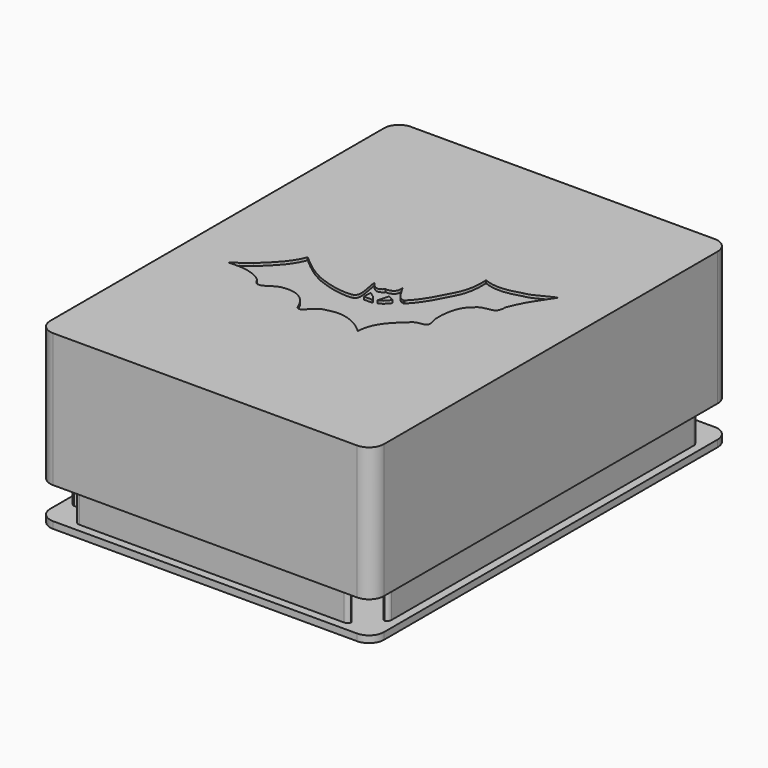
from build123d import *

# Parameters (mm, degrees)
F1_W        = 1.5
F1_H        = 85.4
F1_W_2      = 60.4
F1_H_2      = 1.5
F2_DEPTH    = 1.5
F3_DEPTH    = 29.5
F4_T1_DEPTH = 30.5
F5_DEPTH    = 29.5
F7_T        = -1.5
F9_DEPTH    = 0.6


# Not quite as in the source:
# - a fillet or chamfer that OpenCascade refuses, or shapes differently, is made with other operations: its cross-section is extruded or revolved along the edge and cut away or added


with BuildPart() as f2:
    # F1 (on Top) → F2 (new body)
    with BuildSketch(Plane.XY):
        with BuildLine():
            Line((-35, -46), (-35, -43.0606123087))
            ThreePointArc((-35, -43.0606123087), (-36.3142494559, -44.276631206), (-36.8, -46))
            ThreePointArc((-36.8, -46), (-35.8334523867, -48.3334523691), (-33.5000000248, -49.3))
            ThreePointArc((-33.5000000248, -49.3), (-31.7766312166, -48.8142494624), (-30.5606123087, -47.5))
            Line((-30.5606123087, -47.5), (-33.5000000271, -47.5))
            Line((-33.5000000271, -47.5), (-35, -47.5))
            Line((-35, -47.5), (-35, -46))
        make_face()
        with BuildLine():
            ThreePointArc((33.5, 42.7), (31.1665476221, 43.6665476221), (30.2, 46))
            Line((30.2, 46), (-30.2, 46))
            ThreePointArc((-30.2, 46), (-31.1665476221, 43.6665476221), (-33.5, 42.7))
            Line((-33.5, 42.7), (-33.5, -42.7))
            ThreePointArc((-33.5, -42.7), (-31.1665476221, -43.6665476221), (-30.2, -46))
            Line((-30.2, -46), (30.2, -46))
            ThreePointArc((30.2, -46), (31.1665476221, -43.6665476221), (33.5, -42.7))
            Line((33.5, -42.7), (33.5, 42.7))
        make_face()
        with Locations((34.25, 0)):
            Rectangle(F1_W, F1_H)
        with Locations((-34.25, 0)):
            Rectangle(F1_W, F1_H)
        with BuildLine():
            ThreePointArc((36.8, 46), (36.3142494559, 44.276631206), (35, 43.0606123087))
            Line((35, 43.0606123087), (35, 42.7))
            Line((35, 42.7), (35, -42.7))
            Line((35, -42.7), (35, -43.0606123087))
            ThreePointArc((35, -43.0606123087), (36.3142494559, -44.276631206), (36.8, -46))
            Line((36.8, -46), (36.8, 46))
        make_face()
        with BuildLine():
            ThreePointArc((33.5, -49.3), (31.776631206, -48.8142494559), (30.5606123087, -47.5))
            Line((30.5606123087, -47.5), (30.2, -47.5))
            Line((30.2, -47.5), (-30.2, -47.5))
            Line((-30.2, -47.5), (-30.5606123087, -47.5))
            ThreePointArc((-30.5606123087, -47.5), (-31.7766312166, -48.8142494624), (-33.5000000248, -49.3))
            Line((-33.5000000248, -49.3), (33.5, -49.3))
        make_face()
        with Locations((0, 46.75)):
            Rectangle(F1_W_2, F1_H_2)
        with BuildLine():
            Line((32, 46), (30.2, 46))
            ThreePointArc((30.2, 46), (31.1665476221, 43.6665476221), (33.5, 42.7))
            Line((33.5, 42.7), (33.5, 44.5))
            ThreePointArc((33.5, 44.5), (32.4393398282, 44.9393398282), (32, 46))
        make_face()
        with BuildLine():
            ThreePointArc((33.5, 49.3), (31.776631206, 48.8142494559), (30.5606123087, 47.5))
            Line((30.5606123087, 47.5), (33.5, 47.5))
            Line((33.5, 47.5), (35, 47.5))
            Line((35, 47.5), (35, 46))
            Line((35, 46), (35, 43.0606123087))
            ThreePointArc((35, 43.0606123087), (36.3142494559, 44.276631206), (36.8, 46))
            ThreePointArc((36.8, 46), (35.8334523779, 48.3334523779), (33.5, 49.3))
        make_face()
        with Locations((0, -46.75)):
            Rectangle(F1_W_2, F1_H_2)
        with BuildLine():
            Line((-33.4999999666, 47.5), (-30.5606123087, 47.5))
            ThreePointArc((-30.5606123087, 47.5), (-31.776631206, 48.8142494559), (-33.5, 49.3))
            ThreePointArc((-33.5, 49.3), (-35.8334523779, 48.3334523779), (-36.8, 46))
            ThreePointArc((-36.8, 46), (-36.3142494559, 44.276631206), (-35, 43.0606123087))
            Line((-35, 43.0606123087), (-35, 46))
            Line((-35, 46), (-35, 47.5))
            Line((-35, 47.5), (-33.4999999666, 47.5))
        make_face()
        with BuildLine():
            Line((33.5, -44.5), (33.5, -42.7))
            ThreePointArc((33.5, -42.7), (31.1665476221, -43.6665476221), (30.2, -46))
            Line((30.2, -46), (32, -46))
            ThreePointArc((32, -46), (32.4393398282, -44.9393398282), (33.5, -44.5))
        make_face()
        with BuildLine():
            Line((-35, 42.7), (-35, 43.0606123087))
            ThreePointArc((-35, 43.0606123087), (-36.3142494559, 44.276631206), (-36.8, 46))
            Line((-36.8, 46), (-36.8, -46))
            ThreePointArc((-36.8, -46), (-36.3142494559, -44.276631206), (-35, -43.0606123087))
            Line((-35, -43.0606123087), (-35, -42.7))
            Line((-35, -42.7), (-35, 42.7))
        make_face()
        with BuildLine():
            ThreePointArc((-33.5, 42.7), (-31.1665476221, 43.6665476221), (-30.2, 46))
            Line((-30.2, 46), (-32, 46))
            ThreePointArc((-32, 46), (-32.4393398282, 44.9393398282), (-33.5, 44.5))
            Line((-33.5, 44.5), (-33.5, 42.7))
        make_face()
        with BuildLine():
            ThreePointArc((-30.2, -46), (-31.1665476221, -43.6665476221), (-33.5, -42.7))
            Line((-33.5, -42.7), (-33.5, -44.5))
            ThreePointArc((-33.5, -44.5), (-32.4393398282, -44.9393398282), (-32, -46))
            Line((-32, -46), (-30.2, -46))
        make_face()
        with BuildLine():
            Line((30.2, 47.5), (30.5606123087, 47.5))
            ThreePointArc((30.5606123087, 47.5), (31.776631206, 48.8142494559), (33.5, 49.3))
            Line((33.5, 49.3), (-33.5, 49.3))
            ThreePointArc((-33.5, 49.3), (-31.776631206, 48.8142494559), (-30.5606123087, 47.5))
            Line((-30.5606123087, 47.5), (-30.2, 47.5))
            Line((-30.2, 47.5), (30.2, 47.5))
        make_face()
        with BuildLine():
            Line((-32, 46), (-30.2, 46))
            ThreePointArc((-30.2, 46), (-30.2914193651, 46.7713691135), (-30.5606123087, 47.5))
            Line((-30.5606123087, 47.5), (-33.4999999666, 47.5))
            ThreePointArc((-33.4999999666, 47.5), (-32.4393398164, 47.06066016), (-32, 46))
        make_face()
        with BuildLine():
            ThreePointArc((36.8, -46), (36.3142494559, -44.276631206), (35, -43.0606123087))
            Line((35, -43.0606123087), (35, -46))
            Line((35, -46), (35, -47.5))
            Line((35, -47.5), (33.5, -47.5))
            Line((33.5, -47.5), (30.5606123087, -47.5))
            ThreePointArc((30.5606123087, -47.5), (31.776631206, -48.8142494559), (33.5, -49.3))
            ThreePointArc((33.5, -49.3), (35.8334523779, -48.3334523779), (36.8, -46))
        make_face()
        with BuildLine():
            ThreePointArc((33.5, 47.5), (32.4393398282, 47.0606601718), (32, 46))
            Line((32, 46), (33.5, 46))
            Line((33.5, 46), (33.5, 44.5))
            ThreePointArc((33.5, 44.5), (34.5606601718, 44.9393398282), (35, 46))
            ThreePointArc((35, 46), (34.5606601718, 47.0606601718), (33.5, 47.5))
        make_face()
        with BuildLine():
            ThreePointArc((-30.5606123087, -47.5), (-30.2914193651, -46.7713691135), (-30.2, -46))
            Line((-30.2, -46), (-32, -46))
            ThreePointArc((-32, -46), (-32.4393398378, -47.0606601813), (-33.5000000271, -47.5))
            Line((-33.5000000271, -47.5), (-30.5606123087, -47.5))
        make_face()
        with BuildLine():
            ThreePointArc((35, -43.0606123087), (34.2713691135, -42.7914193651), (33.5, -42.7))
            Line((33.5, -42.7), (33.5, -44.5))
            ThreePointArc((33.5, -44.5), (34.5606601718, -44.9393398282), (35, -46))
            Line((35, -46), (35, -43.0606123087))
        make_face()
        with BuildLine():
            ThreePointArc((30.5606123087, 47.5), (30.2914193651, 46.7713691135), (30.2, 46))
            Line((30.2, 46), (32, 46))
            ThreePointArc((32, 46), (32.4393398282, 47.0606601718), (33.5, 47.5))
            Line((33.5, 47.5), (30.5606123087, 47.5))
        make_face()
        with BuildLine():
            Line((-33.5, 46), (-32, 46))
            ThreePointArc((-32, 46), (-32.4393398164, 47.06066016), (-33.4999999666, 47.5))
            ThreePointArc((-33.4999999666, 47.5), (-34.56066016, 47.0606601836), (-35, 46))
            ThreePointArc((-35, 46), (-34.5606601718, 44.9393398282), (-33.5, 44.5))
            Line((-33.5, 44.5), (-33.5, 46))
        make_face()
        with BuildLine():
            Line((32, -46), (30.2, -46))
            ThreePointArc((30.2, -46), (30.2914193651, -46.7713691135), (30.5606123087, -47.5))
            Line((30.5606123087, -47.5), (33.5, -47.5))
            ThreePointArc((33.5, -47.5), (32.4393398282, -47.0606601718), (32, -46))
        make_face()
        with BuildLine():
            ThreePointArc((35, 43.0606123087), (34.2713691135, 42.7914193651), (33.5, 42.7))
            Line((33.5, 42.7), (35, 42.7))
            Line((35, 42.7), (35, 43.0606123087))
        make_face()
        with BuildLine():
            ThreePointArc((-32, -46), (-32.4393398282, -44.9393398282), (-33.5, -44.5))
            Line((-33.5, -44.5), (-33.5, -46))
            Line((-33.5, -46), (-32, -46))
        make_face()
        with BuildLine():
            Line((33.5, -46), (33.5, -44.5))
            ThreePointArc((33.5, -44.5), (32.4393398282, -44.9393398282), (32, -46))
            Line((32, -46), (33.5, -46))
        make_face()
        with BuildLine():
            Line((-33.5, -44.5), (-33.5, -42.7))
            ThreePointArc((-33.5, -42.7), (-34.2713691135, -42.7914193651), (-35, -43.0606123087))
            Line((-35, -43.0606123087), (-35, -46))
            ThreePointArc((-35, -46), (-34.5606601718, -44.9393398282), (-33.5, -44.5))
        make_face()
        with BuildLine():
            ThreePointArc((-35, 43.0606123087), (-34.2713691135, 42.7914193651), (-33.5, 42.7))
            Line((-33.5, 42.7), (-33.5, 44.5))
            ThreePointArc((-33.5, 44.5), (-34.5606601718, 44.9393398282), (-35, 46))
            Line((-35, 46), (-35, 43.0606123087))
        make_face()
        with BuildLine():
            Line((-33.5, -46), (-33.5, -44.5))
            ThreePointArc((-33.5, -44.5), (-34.5606601718, -44.9393398282), (-35, -46))
            ThreePointArc((-35, -46), (-34.5606601813, -47.0606601622), (-33.5000000271, -47.5))
            ThreePointArc((-33.5000000271, -47.5), (-32.4393398378, -47.0606601813), (-32, -46))
            Line((-32, -46), (-33.5, -46))
        make_face()
        with BuildLine():
            Line((33.5, 44.5), (33.5, 42.7))
            ThreePointArc((33.5, 42.7), (34.2713691135, 42.7914193651), (35, 43.0606123087))
            Line((35, 43.0606123087), (35, 46))
            ThreePointArc((35, 46), (34.5606601718, 44.9393398282), (33.5, 44.5))
        make_face()
        with BuildLine():
            Line((-30.2, -47.5), (-30.2, -46))
            ThreePointArc((-30.2, -46), (-30.2914193651, -46.7713691135), (-30.5606123087, -47.5))
            Line((-30.5606123087, -47.5), (-30.2, -47.5))
        make_face()
        with BuildLine():
            ThreePointArc((-30.5606123087, 47.5), (-30.2914193651, 46.7713691135), (-30.2, 46))
            Line((-30.2, 46), (-30.2, 47.5))
            Line((-30.2, 47.5), (-30.5606123087, 47.5))
        make_face()
        with BuildLine():
            Line((30.2, 47.5), (30.2, 46))
            ThreePointArc((30.2, 46), (30.2914193651, 46.7713691135), (30.5606123087, 47.5))
            Line((30.5606123087, 47.5), (30.2, 47.5))
        make_face()
        with BuildLine():
            ThreePointArc((-35, -43.0606123087), (-34.2713691135, -42.7914193651), (-33.5, -42.7))
            Line((-33.5, -42.7), (-35, -42.7))
            Line((-35, -42.7), (-35, -43.0606123087))
        make_face()
        with BuildLine():
            Line((33.5, 46), (32, 46))
            ThreePointArc((32, 46), (32.4393398282, 44.9393398282), (33.5, 44.5))
            Line((33.5, 44.5), (33.5, 46))
        make_face()
        with BuildLine():
            ThreePointArc((-35, 46), (-34.56066016, 47.0606601836), (-33.4999999666, 47.5))
            Line((-33.4999999666, 47.5), (-35, 47.5))
            Line((-35, 47.5), (-35, 46))
        make_face()
        with BuildLine():
            ThreePointArc((-33.5000000271, -47.5), (-34.5606601813, -47.0606601622), (-35, -46))
            Line((-35, -46), (-35, -47.5))
            Line((-35, -47.5), (-33.5000000271, -47.5))
        make_face()
        with BuildLine():
            Line((35, 47.5), (33.5, 47.5))
            ThreePointArc((33.5, 47.5), (34.5606601718, 47.0606601718), (35, 46))
            Line((35, 46), (35, 47.5))
        make_face()
        with BuildLine():
            Line((35, -47.5), (35, -46))
            ThreePointArc((35, -46), (34.5606601718, -47.0606601718), (33.5, -47.5))
            Line((33.5, -47.5), (35, -47.5))
        make_face()
        with BuildLine():
            Line((-35, 42.7), (-33.5, 42.7))
            ThreePointArc((-33.5, 42.7), (-34.2713691135, 42.7914193651), (-35, 43.0606123087))
            Line((-35, 43.0606123087), (-35, 42.7))
        make_face()
        with BuildLine():
            ThreePointArc((35, -46), (34.5606601718, -44.9393398282), (33.5, -44.5))
            Line((33.5, -44.5), (33.5, -46))
            Line((33.5, -46), (32, -46))
            ThreePointArc((32, -46), (32.4393398282, -47.0606601718), (33.5, -47.5))
            ThreePointArc((33.5, -47.5), (34.5606601718, -47.0606601718), (35, -46))
        make_face()
        with BuildLine():
            Line((35, -42.7), (33.5, -42.7))
            ThreePointArc((33.5, -42.7), (34.2713691135, -42.7914193651), (35, -43.0606123087))
            Line((35, -43.0606123087), (35, -42.7))
        make_face()
        with BuildLine():
            ThreePointArc((30.5606123087, -47.5), (30.2914193651, -46.7713691135), (30.2, -46))
            Line((30.2, -46), (30.2, -47.5))
            Line((30.2, -47.5), (30.5606123087, -47.5))
        make_face()
        with BuildLine():
            ThreePointArc((-33.5, 44.5), (-32.4393398282, 44.9393398282), (-32, 46))
            Line((-32, 46), (-33.5, 46))
            Line((-33.5, 46), (-33.5, 44.5))
        make_face()
    extrude(amount=F2_DEPTH)

    # F1 (on Top) → F3 (join)
    with BuildSketch(Plane.XY):
        with Locations((-34.25, 0)):
            Rectangle(F1_W, F1_H)
        with Locations((0, 46.75)):
            Rectangle(F1_W_2, F1_H_2)
        with Locations((34.25, 0)):
            Rectangle(F1_W, F1_H)
        with Locations((0, -46.75)):
            Rectangle(F1_W_2, F1_H_2)
    extrude(amount=F3_DEPTH)

    # F4: fillet of radius 1 on 16 edges, made by hand

    # F4_s2 → F4_t1 (cut)
    with BuildSketch(Plane.XY.offset(1.5)):
        with BuildLine():
            ThreePointArc((33.5, -41.7), (33.7928932188, -42.4071067812), (34.5, -42.7))
            Line((34.5, -42.7), (33.5, -42.7))
            Line((33.5, -42.7), (33.5, -41.7))
        make_face()
        with BuildLine():
            ThreePointArc((34, -42.7), (34.7071067812, -42.4071067812), (35, -41.7))
            Line((35, -41.7), (35, -42.7))
            Line((35, -42.7), (34, -42.7))
        make_face()
        with BuildLine():
            ThreePointArc((30.2, -47), (29.9071067812, -46.2928932188), (29.2, -46))
            Line((29.2, -46), (30.2, -46))
            Line((30.2, -46), (30.2, -47))
        make_face()
        with BuildLine():
            ThreePointArc((30.2, -46.5), (29.9071067812, -47.2071067812), (29.2, -47.5))
            Line((29.2, -47.5), (30.2, -47.5))
            Line((30.2, -47.5), (30.2, -46.5))
        make_face()
        with BuildLine():
            ThreePointArc((-30.2, -46.5), (-29.9071067812, -47.2071067812), (-29.2, -47.5))
            Line((-29.2, -47.5), (-30.2, -47.5))
            Line((-30.2, -47.5), (-30.2, -46.5))
        make_face()
        with BuildLine():
            ThreePointArc((-29.2, -46), (-29.9071067812, -46.2928932188), (-30.2, -47))
            Line((-30.2, -47), (-30.2, -46))
            Line((-30.2, -46), (-29.2, -46))
        make_face()
        with BuildLine():
            ThreePointArc((-35, -41.7), (-34.7071067812, -42.4071067812), (-34, -42.7))
            Line((-34, -42.7), (-35, -42.7))
            Line((-35, -42.7), (-35, -41.7))
        make_face()
        with BuildLine():
            ThreePointArc((-34.5, -42.7), (-33.7928932188, -42.4071067812), (-33.5, -41.7))
            Line((-33.5, -41.7), (-33.5, -42.7))
            Line((-33.5, -42.7), (-34.5, -42.7))
        make_face()
        with BuildLine():
            ThreePointArc((-34, 42.7), (-34.7071067812, 42.4071067812), (-35, 41.7))
            Line((-35, 41.7), (-35, 42.7))
            Line((-35, 42.7), (-34, 42.7))
        make_face()
        with BuildLine():
            ThreePointArc((-34.5, 42.7), (-33.7928932188, 42.4071067812), (-33.5, 41.7))
            Line((-33.5, 41.7), (-33.5, 42.7))
            Line((-33.5, 42.7), (-34.5, 42.7))
        make_face()
        with BuildLine():
            ThreePointArc((-30.2, 47), (-29.9071067812, 46.2928932188), (-29.2, 46))
            Line((-29.2, 46), (-30.2, 46))
            Line((-30.2, 46), (-30.2, 47))
        make_face()
        with BuildLine():
            ThreePointArc((-29.2, 47.5), (-29.9071067812, 47.2071067812), (-30.2, 46.5))
            Line((-30.2, 46.5), (-30.2, 47.5))
            Line((-30.2, 47.5), (-29.2, 47.5))
        make_face()
        with BuildLine():
            ThreePointArc((30.2, 46.5), (29.9071067812, 47.2071067812), (29.2, 47.5))
            Line((29.2, 47.5), (30.2, 47.5))
            Line((30.2, 47.5), (30.2, 46.5))
        make_face()
        with BuildLine():
            ThreePointArc((30.2, 47), (29.9071067812, 46.2928932188), (29.2, 46))
            Line((29.2, 46), (30.2, 46))
            Line((30.2, 46), (30.2, 47))
        make_face()
        with BuildLine():
            ThreePointArc((33.5, 41.7), (33.7928932188, 42.4071067812), (34.5, 42.7))
            Line((34.5, 42.7), (33.5, 42.7))
            Line((33.5, 42.7), (33.5, 41.7))
        make_face()
        with BuildLine():
            ThreePointArc((35, 41.7), (34.7071067812, 42.4071067812), (34, 42.7))
            Line((34, 42.7), (35, 42.7))
            Line((35, 42.7), (35, 41.7))
        make_face()
    extrude(amount=F4_T1_DEPTH, mode=Mode.SUBTRACT)


with BuildPart() as f5:
    # F1 (on Top) → F5 (new body)
    with BuildSketch(Plane.XY):
        with BuildLine():
            ThreePointArc((33.5, 42.7), (31.1665476221, 43.6665476221), (30.2, 46))
            Line((30.2, 46), (-30.2, 46))
            ThreePointArc((-30.2, 46), (-31.1665476221, 43.6665476221), (-33.5, 42.7))
            Line((-33.5, 42.7), (-33.5, -42.7))
            ThreePointArc((-33.5, -42.7), (-31.1665476221, -43.6665476221), (-30.2, -46))
            Line((-30.2, -46), (30.2, -46))
            ThreePointArc((30.2, -46), (31.1665476221, -43.6665476221), (33.5, -42.7))
            Line((33.5, -42.7), (33.5, 42.7))
        make_face()
        with BuildLine():
            Line((-33.4999999666, 47.5), (-30.5606123087, 47.5))
            ThreePointArc((-30.5606123087, 47.5), (-31.776631206, 48.8142494559), (-33.5, 49.3))
            ThreePointArc((-33.5, 49.3), (-35.8334523779, 48.3334523779), (-36.8, 46))
            ThreePointArc((-36.8, 46), (-36.3142494559, 44.276631206), (-35, 43.0606123087))
            Line((-35, 43.0606123087), (-35, 46))
            Line((-35, 46), (-35, 47.5))
            Line((-35, 47.5), (-33.4999999666, 47.5))
        make_face()
        with BuildLine():
            ThreePointArc((33.5, -49.3), (31.776631206, -48.8142494559), (30.5606123087, -47.5))
            Line((30.5606123087, -47.5), (30.2, -47.5))
            Line((30.2, -47.5), (-30.2, -47.5))
            Line((-30.2, -47.5), (-30.5606123087, -47.5))
            ThreePointArc((-30.5606123087, -47.5), (-31.7766312166, -48.8142494624), (-33.5000000248, -49.3))
            Line((-33.5000000248, -49.3), (33.5, -49.3))
        make_face()
        with BuildLine():
            Line((32, 46), (30.2, 46))
            ThreePointArc((30.2, 46), (31.1665476221, 43.6665476221), (33.5, 42.7))
            Line((33.5, 42.7), (33.5, 44.5))
            ThreePointArc((33.5, 44.5), (32.4393398282, 44.9393398282), (32, 46))
        make_face()
        with Locations((0, 46.75)):
            Rectangle(F1_W_2, F1_H_2)
        with BuildLine():
            Line((-35, -46), (-35, -43.0606123087))
            ThreePointArc((-35, -43.0606123087), (-36.3142494559, -44.276631206), (-36.8, -46))
            ThreePointArc((-36.8, -46), (-35.8334523867, -48.3334523691), (-33.5000000248, -49.3))
            ThreePointArc((-33.5000000248, -49.3), (-31.7766312166, -48.8142494624), (-30.5606123087, -47.5))
            Line((-30.5606123087, -47.5), (-33.5000000271, -47.5))
            Line((-33.5000000271, -47.5), (-35, -47.5))
            Line((-35, -47.5), (-35, -46))
        make_face()
        with Locations((0, -46.75)):
            Rectangle(F1_W_2, F1_H_2)
        with BuildLine():
            ThreePointArc((33.5, 49.3), (31.776631206, 48.8142494559), (30.5606123087, 47.5))
            Line((30.5606123087, 47.5), (33.5, 47.5))
            Line((33.5, 47.5), (35, 47.5))
            Line((35, 47.5), (35, 46))
            Line((35, 46), (35, 43.0606123087))
            ThreePointArc((35, 43.0606123087), (36.3142494559, 44.276631206), (36.8, 46))
            ThreePointArc((36.8, 46), (35.8334523779, 48.3334523779), (33.5, 49.3))
        make_face()
        with BuildLine():
            Line((33.5, -44.5), (33.5, -42.7))
            ThreePointArc((33.5, -42.7), (31.1665476221, -43.6665476221), (30.2, -46))
            Line((30.2, -46), (32, -46))
            ThreePointArc((32, -46), (32.4393398282, -44.9393398282), (33.5, -44.5))
        make_face()
        with BuildLine():
            Line((-35, 42.7), (-35, 43.0606123087))
            ThreePointArc((-35, 43.0606123087), (-36.3142494559, 44.276631206), (-36.8, 46))
            Line((-36.8, 46), (-36.8, -46))
            ThreePointArc((-36.8, -46), (-36.3142494559, -44.276631206), (-35, -43.0606123087))
            Line((-35, -43.0606123087), (-35, -42.7))
            Line((-35, -42.7), (-35, 42.7))
        make_face()
        with Locations((-34.25, 0)):
            Rectangle(F1_W, F1_H)
        with BuildLine():
            ThreePointArc((-33.5, 42.7), (-31.1665476221, 43.6665476221), (-30.2, 46))
            Line((-30.2, 46), (-32, 46))
            ThreePointArc((-32, 46), (-32.4393398282, 44.9393398282), (-33.5, 44.5))
            Line((-33.5, 44.5), (-33.5, 42.7))
        make_face()
        with BuildLine():
            ThreePointArc((36.8, 46), (36.3142494559, 44.276631206), (35, 43.0606123087))
            Line((35, 43.0606123087), (35, 42.7))
            Line((35, 42.7), (35, -42.7))
            Line((35, -42.7), (35, -43.0606123087))
            ThreePointArc((35, -43.0606123087), (36.3142494559, -44.276631206), (36.8, -46))
            Line((36.8, -46), (36.8, 46))
        make_face()
        with BuildLine():
            ThreePointArc((-30.2, -46), (-31.1665476221, -43.6665476221), (-33.5, -42.7))
            Line((-33.5, -42.7), (-33.5, -44.5))
            ThreePointArc((-33.5, -44.5), (-32.4393398282, -44.9393398282), (-32, -46))
            Line((-32, -46), (-30.2, -46))
        make_face()
        with Locations((34.25, 0)):
            Rectangle(F1_W, F1_H)
        with BuildLine():
            Line((30.2, 47.5), (30.5606123087, 47.5))
            ThreePointArc((30.5606123087, 47.5), (31.776631206, 48.8142494559), (33.5, 49.3))
            Line((33.5, 49.3), (-33.5, 49.3))
            ThreePointArc((-33.5, 49.3), (-31.776631206, 48.8142494559), (-30.5606123087, 47.5))
            Line((-30.5606123087, 47.5), (-30.2, 47.5))
            Line((-30.2, 47.5), (30.2, 47.5))
        make_face()
        with BuildLine():
            ThreePointArc((36.8, -46), (36.3142494559, -44.276631206), (35, -43.0606123087))
            Line((35, -43.0606123087), (35, -46))
            Line((35, -46), (35, -47.5))
            Line((35, -47.5), (33.5, -47.5))
            Line((33.5, -47.5), (30.5606123087, -47.5))
            ThreePointArc((30.5606123087, -47.5), (31.776631206, -48.8142494559), (33.5, -49.3))
            ThreePointArc((33.5, -49.3), (35.8334523779, -48.3334523779), (36.8, -46))
        make_face()
        with BuildLine():
            Line((-33.5, -44.5), (-33.5, -42.7))
            ThreePointArc((-33.5, -42.7), (-34.2713691135, -42.7914193651), (-35, -43.0606123087))
            Line((-35, -43.0606123087), (-35, -46))
            ThreePointArc((-35, -46), (-34.5606601718, -44.9393398282), (-33.5, -44.5))
        make_face()
        with BuildLine():
            ThreePointArc((35, -43.0606123087), (34.2713691135, -42.7914193651), (33.5, -42.7))
            Line((33.5, -42.7), (33.5, -44.5))
            ThreePointArc((33.5, -44.5), (34.5606601718, -44.9393398282), (35, -46))
            Line((35, -46), (35, -43.0606123087))
        make_face()
        with BuildLine():
            ThreePointArc((-30.5606123087, -47.5), (-30.2914193651, -46.7713691135), (-30.2, -46))
            Line((-30.2, -46), (-32, -46))
            ThreePointArc((-32, -46), (-32.4393398378, -47.0606601813), (-33.5000000271, -47.5))
            Line((-33.5000000271, -47.5), (-30.5606123087, -47.5))
        make_face()
        with BuildLine():
            ThreePointArc((-35, 43.0606123087), (-34.2713691135, 42.7914193651), (-33.5, 42.7))
            Line((-33.5, 42.7), (-33.5, 44.5))
            ThreePointArc((-33.5, 44.5), (-34.5606601718, 44.9393398282), (-35, 46))
            Line((-35, 46), (-35, 43.0606123087))
        make_face()
        with BuildLine():
            Line((33.5, 46), (32, 46))
            ThreePointArc((32, 46), (32.4393398282, 44.9393398282), (33.5, 44.5))
            Line((33.5, 44.5), (33.5, 46))
        make_face()
        with BuildLine():
            Line((32, -46), (30.2, -46))
            ThreePointArc((30.2, -46), (30.2914193651, -46.7713691135), (30.5606123087, -47.5))
            Line((30.5606123087, -47.5), (33.5, -47.5))
            ThreePointArc((33.5, -47.5), (32.4393398282, -47.0606601718), (32, -46))
        make_face()
        with BuildLine():
            ThreePointArc((-33.5, 44.5), (-32.4393398282, 44.9393398282), (-32, 46))
            Line((-32, 46), (-33.5, 46))
            Line((-33.5, 46), (-33.5, 44.5))
        make_face()
        with BuildLine():
            ThreePointArc((-32, -46), (-32.4393398282, -44.9393398282), (-33.5, -44.5))
            Line((-33.5, -44.5), (-33.5, -46))
            Line((-33.5, -46), (-32, -46))
        make_face()
        with BuildLine():
            ThreePointArc((-30.5606123087, 47.5), (-30.2914193651, 46.7713691135), (-30.2, 46))
            Line((-30.2, 46), (-30.2, 47.5))
            Line((-30.2, 47.5), (-30.5606123087, 47.5))
        make_face()
        with BuildLine():
            ThreePointArc((33.5, 47.5), (32.4393398282, 47.0606601718), (32, 46))
            Line((32, 46), (33.5, 46))
            Line((33.5, 46), (33.5, 44.5))
            ThreePointArc((33.5, 44.5), (34.5606601718, 44.9393398282), (35, 46))
            ThreePointArc((35, 46), (34.5606601718, 47.0606601718), (33.5, 47.5))
        make_face()
        with BuildLine():
            ThreePointArc((30.5606123087, 47.5), (30.2914193651, 46.7713691135), (30.2, 46))
            Line((30.2, 46), (32, 46))
            ThreePointArc((32, 46), (32.4393398282, 47.0606601718), (33.5, 47.5))
            Line((33.5, 47.5), (30.5606123087, 47.5))
        make_face()
        with BuildLine():
            Line((-33.5, 46), (-32, 46))
            ThreePointArc((-32, 46), (-32.4393398164, 47.06066016), (-33.4999999666, 47.5))
            ThreePointArc((-33.4999999666, 47.5), (-34.56066016, 47.0606601836), (-35, 46))
            ThreePointArc((-35, 46), (-34.5606601718, 44.9393398282), (-33.5, 44.5))
            Line((-33.5, 44.5), (-33.5, 46))
        make_face()
        with BuildLine():
            Line((33.5, 44.5), (33.5, 42.7))
            ThreePointArc((33.5, 42.7), (34.2713691135, 42.7914193651), (35, 43.0606123087))
            Line((35, 43.0606123087), (35, 46))
            ThreePointArc((35, 46), (34.5606601718, 44.9393398282), (33.5, 44.5))
        make_face()
        with BuildLine():
            Line((-30.2, -47.5), (-30.2, -46))
            ThreePointArc((-30.2, -46), (-30.2914193651, -46.7713691135), (-30.5606123087, -47.5))
            Line((-30.5606123087, -47.5), (-30.2, -47.5))
        make_face()
        with BuildLine():
            Line((-32, 46), (-30.2, 46))
            ThreePointArc((-30.2, 46), (-30.2914193651, 46.7713691135), (-30.5606123087, 47.5))
            Line((-30.5606123087, 47.5), (-33.4999999666, 47.5))
            ThreePointArc((-33.4999999666, 47.5), (-32.4393398164, 47.06066016), (-32, 46))
        make_face()
        with BuildLine():
            Line((-35, 42.7), (-33.5, 42.7))
            ThreePointArc((-33.5, 42.7), (-34.2713691135, 42.7914193651), (-35, 43.0606123087))
            Line((-35, 43.0606123087), (-35, 42.7))
        make_face()
        with BuildLine():
            ThreePointArc((35, -46), (34.5606601718, -44.9393398282), (33.5, -44.5))
            Line((33.5, -44.5), (33.5, -46))
            Line((33.5, -46), (32, -46))
            ThreePointArc((32, -46), (32.4393398282, -47.0606601718), (33.5, -47.5))
            ThreePointArc((33.5, -47.5), (34.5606601718, -47.0606601718), (35, -46))
        make_face()
        with BuildLine():
            Line((33.5, -46), (33.5, -44.5))
            ThreePointArc((33.5, -44.5), (32.4393398282, -44.9393398282), (32, -46))
            Line((32, -46), (33.5, -46))
        make_face()
        with BuildLine():
            ThreePointArc((-35, 46), (-34.56066016, 47.0606601836), (-33.4999999666, 47.5))
            Line((-33.4999999666, 47.5), (-35, 47.5))
            Line((-35, 47.5), (-35, 46))
        make_face()
        with BuildLine():
            ThreePointArc((-33.5000000271, -47.5), (-34.5606601813, -47.0606601622), (-35, -46))
            Line((-35, -46), (-35, -47.5))
            Line((-35, -47.5), (-33.5000000271, -47.5))
        make_face()
        with BuildLine():
            ThreePointArc((-35, -43.0606123087), (-34.2713691135, -42.7914193651), (-33.5, -42.7))
            Line((-33.5, -42.7), (-35, -42.7))
            Line((-35, -42.7), (-35, -43.0606123087))
        make_face()
        with BuildLine():
            Line((30.2, 47.5), (30.2, 46))
            ThreePointArc((30.2, 46), (30.2914193651, 46.7713691135), (30.5606123087, 47.5))
            Line((30.5606123087, 47.5), (30.2, 47.5))
        make_face()
        with BuildLine():
            ThreePointArc((35, 43.0606123087), (34.2713691135, 42.7914193651), (33.5, 42.7))
            Line((33.5, 42.7), (35, 42.7))
            Line((35, 42.7), (35, 43.0606123087))
        make_face()
        with BuildLine():
            Line((-33.5, -46), (-33.5, -44.5))
            ThreePointArc((-33.5, -44.5), (-34.5606601718, -44.9393398282), (-35, -46))
            ThreePointArc((-35, -46), (-34.5606601813, -47.0606601622), (-33.5000000271, -47.5))
            ThreePointArc((-33.5000000271, -47.5), (-32.4393398378, -47.0606601813), (-32, -46))
            Line((-32, -46), (-33.5, -46))
        make_face()
        with BuildLine():
            Line((35, -42.7), (33.5, -42.7))
            ThreePointArc((33.5, -42.7), (34.2713691135, -42.7914193651), (35, -43.0606123087))
            Line((35, -43.0606123087), (35, -42.7))
        make_face()
        with BuildLine():
            ThreePointArc((30.5606123087, -47.5), (30.2914193651, -46.7713691135), (30.2, -46))
            Line((30.2, -46), (30.2, -47.5))
            Line((30.2, -47.5), (30.5606123087, -47.5))
        make_face()
        with BuildLine():
            Line((35, 47.5), (33.5, 47.5))
            ThreePointArc((33.5, 47.5), (34.5606601718, 47.0606601718), (35, 46))
            Line((35, 46), (35, 47.5))
        make_face()
        with BuildLine():
            Line((35, -47.5), (35, -46))
            ThreePointArc((35, -46), (34.5606601718, -47.0606601718), (33.5, -47.5))
            Line((33.5, -47.5), (35, -47.5))
        make_face()
    extrude(amount=-F5_DEPTH)


with BuildPart() as f5_1:
    # F6: moved
    add(f5.part.moved(Location((0, 0, 38))))

    # F7
    f7_openings = [f5_1.faces().sort_by_distance(p)[0] for p in [
        (0, 0, 8.5),
    ]]
    offset(amount=F7_T, openings=f7_openings)

    # F8 (on face) → F9 (cut)
    with BuildSketch(Plane.XY.offset(38)):
        with BuildLine():
            add(Edge.make_bspline(
                [(-22.9413497492, -7.3130649169), (-23.5760616462, -7.8160316014), (-24.2193427536, -8.3005692996), (-24.8729026409, -8.7585814894)],
                knots=[0, 0, 0, 0, 0.5352911654, 0.5352911654, 0.5352911654, 0.5352911654], degree=3))
            add(Edge.make_bspline(
                [(-24.8729026411, -8.7585814887), (-22.7026643795, -8.7642749465), (-20.5124119355, -9.1406888103), (-18.6437879762, -10.5905057519)],
                knots=[0.213352112, 0.213352112, 0.213352112, 0.213352112, 1, 1, 1, 1], degree=3))
            add(Edge.make_bspline(
                [(-18.6437879762, -10.5905057519), (-17.2986563401, -13.584726252), (-15.207783504, -10.1620825166), (-13.2913183591, -10.1913781569)],
                knots=[0, 0, 0, 0, 1, 1, 1, 1], degree=3))
            add(Edge.make_bspline(
                [(-13.2913183591, -10.1913781569), (-10.928368334, -9.7728088138), (-8.4512514483, -10.6665962179), (-7.1764557663, -13.3923592376)],
                knots=[0, 0, 0, 0, 1, 1, 1, 1], degree=3))
            add(Edge.make_bspline(
                [(-7.1764557663, -13.3923592376), (-6.1248129155, -16.2572165505), (-4.2056455468, -11.7421978558), (-2.4649607546, -11.967329217)],
                knots=[0, 0, 0, 0, 1, 1, 1, 1], degree=3))
            add(Edge.make_bspline(
                [(-2.4649607546, -11.967329217), (0.7413286532, -10.8821139879), (4.2669554845, -12.1540254374), (6.8463447953, -14.6603241692)],
                knots=[0, 0, 0, 0, 1, 1, 1, 1], degree=3))
            add(Edge.make_bspline(
                [(6.8463447953, -14.6603241692), (6.7614286154, -11.0187683731), (9.4233627225, -8.6607527357), (11.6044647166, -6.9083753608)],
                knots=[0, 0, 0, 0, 1, 1, 1, 1], degree=3))
            add(Edge.make_bspline(
                [(11.6044647166, -6.9083753608), (12.4576274299, -5.6430832856), (14.8489355829, -6.5551982254), (14.7923400437, -5.1155513342)],
                knots=[0, 0, 0, 0, 0.8539890071, 0.8539890071, 0.8539890071, 0.8539890071], degree=3))
            add(Edge.make_bspline(
                [(14.7923400437, -5.1155513342), (14.7685567702, -5.0488709936), (14.7423586347, -4.9796348512), (14.7136557679, -4.9077341632)],
                knots=[0.9759440179, 0.9759440179, 0.9759440179, 0.9759440179, 1, 1, 1, 1], degree=3))
            add(Edge.make_bspline(
                [(14.7136557679, -4.9077341632), (14.7093228243, -4.8136295296), (14.7055854835, -4.718977197), (14.7024766585, -4.6238546724)],
                knots=[0, 0, 0, 0, 0.0312727725, 0.0312727725, 0.0312727725, 0.0312727725], degree=3))
            add(Edge.make_bspline(
                [(14.7024766585, -4.6238546724), (14.6604436726, -4.481042103), (14.6030519544, -4.3231050197), (14.5287129698, -4.1482384427)],
                knots=[0.9371550745, 0.9371550745, 0.9371550745, 0.9371550745, 1, 1, 1, 1], degree=3))
            add(Edge.make_bspline(
                [(14.5287129698, -4.1482384427), (14.3913534949, -1.3468624585), (14.8577585547, 1.975869383), (16.9948029842, 3.4607399393)],
                knots=[0, 0, 0, 0, 1, 1, 1, 1], degree=3))
            add(Edge.make_bspline(
                [(16.9948029842, 3.4607399393), (18.4260473443, 5.3273074296), (21.3783531448, 3.4471947133), (21.2676993301, 6.7967680239)],
                knots=[0, 0, 0, 0, 1, 1, 1, 1], degree=3))
            add(Edge.make_bspline(
                [(21.2676993301, 6.7967680239), (21.9197881787, 8.7083590316), (22.8593960736, 10.4120351541), (23.909175959, 12.0131593117)],
                knots=[0, 0, 0, 0, 0.5755878955, 0.5755878955, 0.5755878955, 0.5755878955], degree=3))
            add(Edge.make_bspline(
                [(23.909175959, 12.0131593117), (24.5979884284, 13.1664893677), (25.3423202005, 14.2671726276), (26.0900177896, 15.3482060519)],
                knots=[0.5268633096, 0.5268633096, 0.5268633096, 0.5268633096, 0.908526515, 0.908526515, 0.908526515, 0.908526515], degree=3))
            add(Edge.make_bspline(
                [(26.0900177896, 15.3482060519), (24.1488041427, 14.6756091702), (22.4201938233, 13.2136382467), (20.3807777138, 12.9228711234)],
                knots=[0.0409615452, 0.0409615452, 0.0409615452, 0.0409615452, 1, 1, 1, 1], degree=3))
            add(Edge.make_bspline(
                [(20.3807777138, 12.9228711234), (17.7783279601, 12.0454817), (14.9500696375, 11.5889034198), (12.3551491588, 12.707109283)],
                knots=[0, 0, 0, 0, 0.9509269266, 0.9509269266, 0.9509269266, 0.9509269266], degree=3))
            add(Edge.make_bspline(
                [(12.3551491613, 12.707109284), (12.5080946481, 10.2877848219), (12.1768124229, 7.8073871476), (11.0878696102, 5.8105019343)],
                knots=[0.0959141776, 0.0959141776, 0.0959141776, 0.0959141776, 1, 1, 1, 1], degree=3))
            add(Edge.make_bspline(
                [(11.0878696102, 5.8105019343), (9.7046696412, 2.9603522841), (8.1883087988, 0.047422054), (6.1078473532, -1.9507587712)],
                knots=[0, 0, 0, 0, 1, 1, 1, 1], degree=3))
            add(Edge.make_bspline(
                [(6.1078473532, -1.9507587712), (6.0785224722, -1.9497217998), (6.0494810296, -1.9477564387), (6.0207158212, -1.9448895597)],
                knots=[0, 0, 0, 0, 0.019478373, 0.019478373, 0.019478373, 0.019478373], degree=3))
            add(Edge.make_bspline(
                [(6.0207158305, -1.9448895794), (5.9923597567, -1.972669857), (5.9638984363, -2.000280188), (5.9353307535, -2.0277180416)],
                knots=[0.9862685875, 0.9862685875, 0.9862685875, 0.9862685875, 1, 1, 1, 1], degree=3))
            add(Edge.make_bspline(
                [(5.9353307535, -2.0277180416), (4.557001105, -1.9789782264), (3.8048415176, 0.1207563442), (2.9308041535, 1.48119636)],
                knots=[0, 0, 0, 0, 0.9155241101, 0.9155241101, 0.9155241101, 0.9155241101], degree=3))
            add(Edge.make_bspline(
                [(2.9308041469, 1.4811963575), (3.0823948261, 0.3115926561), (2.742426417, -0.2646610524), (2.107063054, -0.5025107188)],
                knots=[0.0721218406, 0.0721218406, 0.0721218406, 0.0721218406, 0.6923701781, 0.6923701781, 0.6923701781, 0.6923701781], degree=3))
            add(Edge.make_bspline(
                [(2.107063054, -0.5025107188), (1.7889331889, -0.6700990442), (1.3755573164, -0.7277049334), (0.8997091796, -0.7179229901)],
                knots=[0.6335885985, 0.6335885985, 0.6335885985, 0.6335885985, 0.9752013664, 0.9752013664, 0.9752013664, 0.9752013664], degree=3))
            add(Edge.make_bspline(
                [(0.8997091804, -0.7179229915), (0.6450331492, -1.0093338269), (0.4022761605, -1.1842492029), (0.1686021387, -1.2664318556)],
                knots=[0.0195076297, 0.0195076297, 0.0195076297, 0.0195076297, 0.2398921319, 0.2398921319, 0.2398921319, 0.2398921319], degree=3))
            add(Edge.make_bspline(
                [(0.1686021387, -1.2664318556), (-0.6486882022, -1.7082175208), (-1.3509786529, -0.9908065101), (-2.0527264064, -0.0731956821)],
                knots=[0.186179007, 0.186179007, 0.186179007, 0.186179007, 0.9421201184, 0.9421201184, 0.9421201184, 0.9421201184], degree=3))
            add(Edge.make_bspline(
                [(-2.0527264111, -0.073195683), (-2.0422849341, -1.9687212292), (-0.5978921576, -5.3144141799), (-2.1083712055, -5.8198549895)],
                knots=[0.0501467191, 0.0501467191, 0.0501467191, 0.0501467191, 0.9884755517, 0.9884755517, 0.9884755517, 0.9884755517], degree=3))
            add(Edge.make_bspline(
                [(-2.1083712055, -5.8198549895), (-2.1766743592, -5.8591634853), (-2.2529539116, -5.8908135266), (-2.3378867836, -5.9141433698)],
                knots=[0.949678724, 0.949678724, 0.949678724, 0.949678724, 1, 1, 1, 1], degree=3))
            add(Edge.make_bspline(
                [(-2.3378867836, -5.9141433698), (-5.1514830825, -6.1905726429), (-7.9773248114, -5.3480698178), (-10.6605427677, -4.2755046546)],
                knots=[0, 0, 0, 0, 1, 1, 1, 1], degree=3))
            add(Edge.make_bspline(
                [(-10.6605427677, -4.2755046546), (-12.9292984467, -3.238663106), (-14.9912757386, -1.5426044276), (-16.9860102536, 0.2072609439)],
                knots=[0, 0, 0, 0, 0.982318537, 0.982318537, 0.982318537, 0.982318537], degree=3))
            add(Edge.make_bspline(
                [(-16.9860102536, 0.2072609439), (-18.266626669, -3.1051039448), (-20.7136822354, -5.2479311393), (-22.9413497492, -7.3130649169)],
                knots=[0.0168646563, 0.0168646563, 0.0168646563, 0.0168646563, 1, 1, 1, 1], degree=3))
        make_face()
        Polygon((1.0385320271, -4.2863696715), (1.6647713738, -5.1971167466), (-0.2922274374, -5.1971167466), (-0.2139457362, -3.3756207361), align=None, mode=Mode.SUBTRACT)
        Polygon((3.3066170999, -4.3504795037), (2.4314863572, -4.8032394963), (3.0950939081, -2.4232727481), (4.3941048016, -3.1361305362), align=None, mode=Mode.SUBTRACT)
        with BuildLine():
            add(Edge.make_bspline(
                [(-24.8729026409, -8.7585814894), (-25.4177434955, -9.1404038101), (-25.9697278348, -9.5037915924), (-26.529846125, -9.8440539883)],
                knots=[0.5352911654, 0.5352911654, 0.5352911654, 0.5352911654, 0.9815371816, 0.9815371816, 0.9815371816, 0.9815371816], degree=3))
            add(Edge.make_bspline(
                [(-26.5298461242, -9.8440539908), (-23.8214921414, -9.6577085095), (-20.9420292861, -9.7946674754), (-18.5744445428, -11.7508731878)],
                knots=[0.0118832165, 0.0118832165, 0.0118832165, 0.0118832165, 1, 1, 1, 1], degree=3))
            add(Edge.make_bspline(
                [(-18.5744445428, -11.7508731878), (-17.9905942896, -13.1348782908), (-17.2674589975, -13.2425683768), (-16.4789913617, -12.9186007484)],
                knots=[0, 0, 0, 0, 0.4303094298, 0.4303094298, 0.4303094298, 0.4303094298], degree=3))
            add(Edge.make_bspline(
                [(-16.4789913617, -12.9186007484), (-15.7475511513, -12.5681518129), (-14.9656711455, -11.9061560676), (-14.19039546, -11.5841484702)],
                knots=[0.4615109586, 0.4615109586, 0.4615109586, 0.4615109586, 0.8561499184, 0.8561499184, 0.8561499184, 0.8561499184], degree=3))
            add(Edge.make_bspline(
                [(-14.19039546, -11.5841484702), (-13.8500305468, -11.422358453), (-13.5101226785, -11.3166921699), (-13.175486445, -11.3221398867)],
                knots=[0.8268924715, 0.8268924715, 0.8268924715, 0.8268924715, 1, 1, 1, 1], degree=3))
            add(Edge.make_bspline(
                [(-13.175486445, -11.3221398867), (-10.7920140924, -10.8725267523), (-8.2933826687, -11.8326043714), (-7.0075145358, -14.7605396175)],
                knots=[0, 0, 0, 0, 1, 1, 1, 1], degree=3))
            add(Edge.make_bspline(
                [(-7.0075145358, -14.7605396175), (-6.6861773534, -15.6927500519), (-6.2845406341, -15.8975204802), (-5.8319337959, -15.736751186)],
                knots=[0, 0, 0, 0, 0.3029265659, 0.3029265659, 0.3029265659, 0.3029265659], degree=3))
            add(Edge.make_bspline(
                [(-5.8319337959, -15.736751186), (-4.9806923478, -15.2850425155), (-3.9709050892, -13.7599764555), (-2.9825924025, -13.3828511365)],
                knots=[0.340891627, 0.340891627, 0.340891627, 0.340891627, 0.895530138, 0.895530138, 0.895530138, 0.895530138], degree=3))
            add(Edge.make_bspline(
                [(-2.9825924025, -13.3828511365), (-2.7385269457, -13.2588548311), (-2.4951304424, -13.196755251), (-2.2550985855, -13.2298149752)],
                knots=[0.8632922845, 0.8632922845, 0.8632922845, 0.8632922845, 1, 1, 1, 1], degree=3))
            add(Edge.make_bspline(
                [(-2.2550985855, -13.2298149752), (0.9074346434, -12.0899168753), (4.3779732355, -13.3711008677), (6.962876718, -15.9456971656)],
                knots=[0, 0, 0, 0, 0.9778598071, 0.9778598071, 0.9778598071, 0.9778598071], degree=3))
            add(Edge.make_bspline(
                [(6.9628767159, -15.9456971667), (6.9957234985, -12.1777513303), (9.611914343, -9.7139198082), (11.764009092, -7.8725929791)],
                knots=[0.0217956059, 0.0217956059, 0.0217956059, 0.0217956059, 1, 1, 1, 1], degree=3))
            add(Edge.make_bspline(
                [(11.764009092, -7.8725929791), (11.962476172, -7.5591452767), (12.2434623184, -7.3700959048), (12.5576501162, -7.2457696467)],
                knots=[0, 0, 0, 0, 0.1969486194, 0.1969486194, 0.1969486194, 0.1969486194], degree=3))
            add(Edge.make_bspline(
                [(12.5576501162, -7.2457696467), (13.1906151748, -6.927999741), (14.0124003821, -6.9479575103), (14.5599827439, -6.7453739897)],
                knots=[0.160105494, 0.160105494, 0.160105494, 0.160105494, 0.5755889685, 0.5755889685, 0.5755889685, 0.5755889685], degree=3))
            add(Edge.make_bspline(
                [(14.5599827439, -6.7453739897), (14.9694064595, -6.5244990451), (15.142292993, -6.0967023023), (14.7923400437, -5.1155513342)],
                knots=[0.6219783681, 0.6219783681, 0.6219783681, 0.6219783681, 0.9759440179, 0.9759440179, 0.9759440179, 0.9759440179], degree=3))
            add(Edge.make_bspline(
                [(11.6044647166, -6.9083753608), (12.4576274299, -5.6430832856), (14.8489355829, -6.5551982254), (14.7923400437, -5.1155513342)],
                knots=[0, 0, 0, 0, 0.8539890071, 0.8539890071, 0.8539890071, 0.8539890071], degree=3))
            add(Edge.make_bspline(
                [(6.8463447953, -14.6603241692), (6.7614286154, -11.0187683731), (9.4233627225, -8.6607527357), (11.6044647166, -6.9083753608)],
                knots=[0, 0, 0, 0, 1, 1, 1, 1], degree=3))
            add(Edge.make_bspline(
                [(-2.4649607546, -11.967329217), (0.7413286532, -10.8821139879), (4.2669554845, -12.1540254374), (6.8463447953, -14.6603241692)],
                knots=[0, 0, 0, 0, 1, 1, 1, 1], degree=3))
            add(Edge.make_bspline(
                [(-7.1764557663, -13.3923592376), (-6.1248129155, -16.2572165505), (-4.2056455468, -11.7421978558), (-2.4649607546, -11.967329217)],
                knots=[0, 0, 0, 0, 1, 1, 1, 1], degree=3))
            add(Edge.make_bspline(
                [(-13.2913183591, -10.1913781569), (-10.928368334, -9.7728088138), (-8.4512514483, -10.6665962179), (-7.1764557663, -13.3923592376)],
                knots=[0, 0, 0, 0, 1, 1, 1, 1], degree=3))
            add(Edge.make_bspline(
                [(-18.6437879762, -10.5905057519), (-17.2986563401, -13.584726252), (-15.207783504, -10.1620825166), (-13.2913183591, -10.1913781569)],
                knots=[0, 0, 0, 0, 1, 1, 1, 1], degree=3))
            add(Edge.make_bspline(
                [(-24.8729026411, -8.7585814887), (-22.7026643795, -8.7642749465), (-20.5124119355, -9.1406888103), (-18.6437879762, -10.5905057519)],
                knots=[0.213352112, 0.213352112, 0.213352112, 0.213352112, 1, 1, 1, 1], degree=3))
        make_face()
    extrude(amount=-F9_DEPTH, mode=Mode.SUBTRACT)


solid = Compound([f2.part, f5_1.part])
